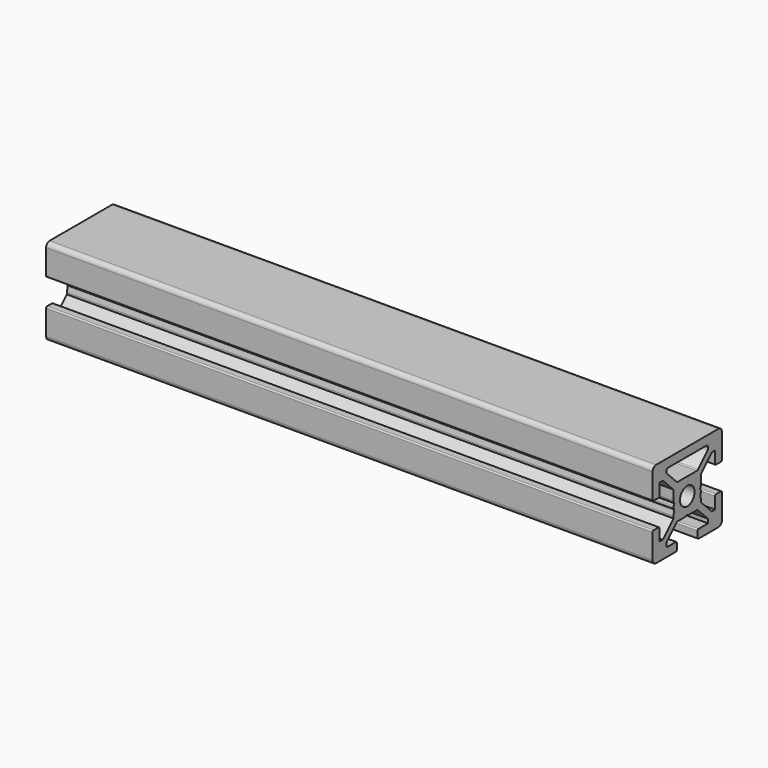
from build123d import *

# Parameters (mm, degrees)
F1_DEPTH = 70


# Not quite as in the source:
# - ends of sketch curves that miss each other by under 0.0002 mm in the source are joined


with BuildPart() as f1:
    # F0 (on Right) → F1 (new body, symmetric)
    with BuildSketch(Plane.YZ):
        with BuildLine():
            Line((9.043565, 10.073321), (0.043565, 10.073321))
            Line((0.043565, 10.073321), (-8.956435, 10.073321))
            ThreePointArc((-8.956435, 10.073321), (-9.6635417812, 9.7804277812), (-9.956435, 9.073321))
            Line((-9.956435, 9.073321), (-9.956435, 3.373321))
            ThreePointArc((-9.956435, 3.373321), (-9.8685670344, 3.1611889656), (-9.656435, 3.073321))
            Line((-9.656435, 3.073321), (-8.256435, 3.073321))
            ThreePointArc((-8.256435, 3.073321), (-8.0443029656, 3.1611889656), (-7.956435, 3.373321))
            Line((-7.956435, 3.373321), (-7.956435, 6.073321))
            Line((-7.956435, 6.073321), (-7.017095, 6.073321))
            Line((-7.017095, 6.073321), (-3.956435, 3.012661))
            Line((-3.956435, 3.012661), (-3.956435, 0.726911))
            ThreePointArc((-3.956435, 0.726911), (-3.9393979324, 0.5975015494), (-3.8894477764, 0.4769111291))
            Line((-3.8894477764, 0.4769111291), (-3.656435, 0.073321))
            Line((-3.656435, 0.073321), (-3.889448, -0.330269))
            ThreePointArc((-3.889448, -0.330269), (-3.956435, -0.580269), (-3.8894477764, -0.8302688709))
            Line((-3.8894477764, -0.8302688709), (-3.707412, -1.145565))
            Line((-3.707412, -1.145565), (-3.956435, -2.426679))
            Line((-3.956435, -2.426679), (-3.956435, -2.866019))
            Line((-3.956435, -2.866019), (-7.017095, -5.926679))
            Line((-7.017095, -5.926679), (-7.956435, -5.926679))
            Line((-7.956435, -5.926679), (-7.956435, -3.226679))
            ThreePointArc((-7.956435, -3.226679), (-8.0443029656, -3.0145469656), (-8.256435, -2.926679))
            Line((-8.256435, -2.926679), (-9.656435, -2.926679))
            ThreePointArc((-9.656435, -2.926679), (-9.8685670344, -3.0145469656), (-9.956435, -3.226679))
            Line((-9.956435, -3.226679), (-9.956435, -8.926679))
            ThreePointArc((-9.956435, -8.926679), (-9.6635417812, -9.6337857812), (-8.956435, -9.926679))
            Line((-8.956435, -9.926679), (-3.256435, -9.926679))
            ThreePointArc((-3.256435, -9.926679), (-3.0443029656, -9.8388110344), (-2.956435, -9.626679))
            Line((-2.956435, -9.626679), (-2.956435, -8.226679))
            ThreePointArc((-2.956435, -8.226679), (-3.0443029656, -8.0145469656), (-3.256435, -7.926679))
            Line((-3.256435, -7.926679), (-5.956435, -7.926679))
            Line((-5.956435, -7.926679), (-5.956435, -6.987339))
            Line((-5.956435, -6.987339), (-2.895775, -3.926679))
            Line((-2.895775, -3.926679), (-0.610025, -3.926679))
            ThreePointArc((-0.610025, -3.926679), (-0.4806155494, -3.9096419324), (-0.3600251291, -3.8596917764))
            Line((-0.3600251291, -3.8596917764), (-0.0645959325, -3.6891257984))
            Line((-0.0645959325, -3.6891257984), (0.2217128734, -3.8544264098))
            ThreePointArc((0.2217128734, -3.8544264098), (0.3921793907, -3.9150473077), (0.5730594828, -3.9110345539))
            ThreePointArc((0.5730594828, -3.9110345539), (0.6346161199, -3.9227524708), (0.697155, -3.926679))
            Line((0.697155, -3.926679), (2.982905, -3.926679))
            Line((2.982905, -3.926679), (6.043565, -6.987339))
            Line((6.043565, -6.987339), (6.043565, -7.926679))
            Line((6.043565, -7.926679), (3.343565, -7.926679))
            ThreePointArc((3.343565, -7.926679), (3.1314329656, -8.0145469656), (3.043565, -8.226679))
            Line((3.043565, -8.226679), (3.043565, -9.626679))
            ThreePointArc((3.043565, -9.626679), (3.1314329656, -9.8388110344), (3.343565, -9.926679))
            Line((3.343565, -9.926679), (9.043565, -9.926679))
            ThreePointArc((9.043565, -9.926679), (9.7506717812, -9.6337857812), (10.043565, -8.926679))
            Line((10.043565, -8.926679), (10.043565, -3.226679))
            ThreePointArc((10.043565, -3.226679), (9.9556970344, -3.0145469656), (9.743565, -2.926679))
            Line((9.743565, -2.926679), (8.343565, -2.926679))
            ThreePointArc((8.343565, -2.926679), (8.1314329656, -3.0145469656), (8.043565, -3.226679))
            Line((8.043565, -3.226679), (8.043565, -5.926679))
            Line((8.043565, -5.926679), (7.104225, -5.926679))
            Line((7.104225, -5.926679), (4.043565, -2.866019))
            Line((4.043565, -2.866019), (4.043565, -2.426679))
            Line((4.043565, -2.426679), (3.794542, -1.145565))
            Line((3.794542, -1.145565), (3.976578, -0.830269))
            ThreePointArc((3.976578, -0.830269), (4.043565, -0.580269), (3.9765777764, -0.3302691291))
            Line((3.9765777764, -0.3302691291), (3.743565, 0.073321))
            Line((3.743565, 0.073321), (3.976578, 0.476911))
            ThreePointArc((3.976578, 0.476911), (4.0265279324, 0.5975015494), (4.043565, 0.726911))
            Line((4.043565, 0.726911), (4.043565, 3.012661))
            Line((4.043565, 3.012661), (7.104225, 6.073321))
            Line((7.104225, 6.073321), (8.043565, 6.073321))
            Line((8.043565, 6.073321), (8.043565, 3.373321))
            ThreePointArc((8.043565, 3.373321), (8.1314329656, 3.1611889656), (8.343565, 3.073321))
            Line((8.343565, 3.073321), (9.743565, 3.073321))
            ThreePointArc((9.743565, 3.073321), (9.9556970344, 3.1611889656), (10.043565, 3.373321))
            Line((10.043565, 3.373321), (10.043565, 9.073321))
            ThreePointArc((10.043565, 9.073321), (9.7506717812, 9.7804277812), (9.043565, 10.073321))
        make_face()
        with BuildLine():
            ThreePointArc((0.043565, 2.173321), (2.143565, 0.073321), (0.043565, -2.026679))
            ThreePointArc((0.043565, -2.026679), (-2.056435, 0.073321), (0.043565, 2.173321))
        make_face(mode=Mode.SUBTRACT)
        with BuildLine():
            Line((2.775798, 4.073321), (0.043565, 4.073321))
            Line((0.043565, 4.073321), (-2.688668, 4.073321))
            ThreePointArc((-2.688668, 4.073321), (-2.8800097162, 4.1113812337), (-3.0422213906, 4.2197676094))
            Line((-3.0422213906, 4.2197676094), (-5.809988, 6.987535))
            ThreePointArc((-5.809988, 6.987535), (-5.9183747663, 7.1497462838), (-5.956435, 7.341088))
            Line((-5.956435, 7.341088), (-5.956435, 7.573321))
            ThreePointArc((-5.956435, 7.573321), (-5.8099883906, 7.9268743906), (-5.456435, 8.073321))
            Line((-5.456435, 8.073321), (0.043565, 8.073321))
            Line((0.043565, 8.073321), (5.543565, 8.073321))
            ThreePointArc((5.543565, 8.073321), (5.8971183906, 7.9268743906), (6.043565, 7.573321))
            Line((6.043565, 7.573321), (6.043565, 7.341088))
            ThreePointArc((6.043565, 7.341088), (6.0055047663, 7.1497462838), (5.8971183906, 6.9875346094))
            Line((5.8971183906, 6.9875346094), (3.129351, 4.219768))
            ThreePointArc((3.129351, 4.219768), (2.9671397162, 4.1113812337), (2.775798, 4.073321))
        make_face(mode=Mode.SUBTRACT)
    extrude(amount=F1_DEPTH, both=True)


solid = f1.part
